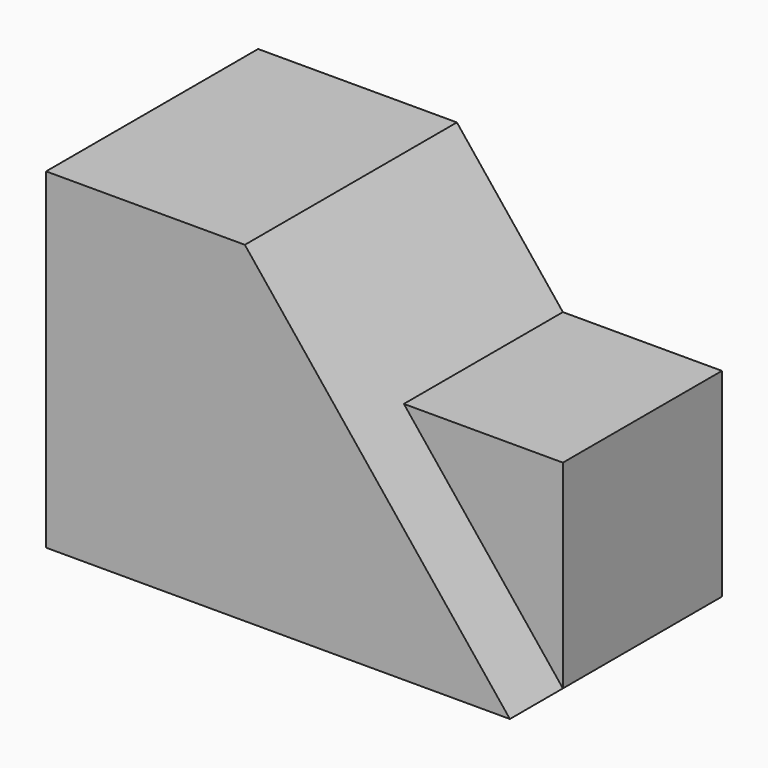
from build123d import *

# Parameters (mm, degrees)
F1_DEPTH = 25.4
F5_DEPTH = 19.05


# Not quite as in the source:
# - a feature of the source that left no trace in its solid (it failed there, or was rolled back) is left out


with BuildPart() as f1:
    # F0 (on Front) → F1 (new body)
    with BuildSketch(Plane.XZ):
        Polygon((0, 31.75), (0, 0), (44.45, 0), (19.05, 31.75), align=None)
    extrude(amount=F1_DEPTH)

    # F4 (on face) → F5 (join)
    with BuildSketch(Plane(origin=(0, 0, 0), x_dir=(-1, 0, 0), z_dir=(0, 1, 0))):
        Polygon((-44.45, 19.05), (-44.45, 0), (-29.21, 19.05), align=None)
    extrude(amount=-F5_DEPTH)


solid = f1.part
